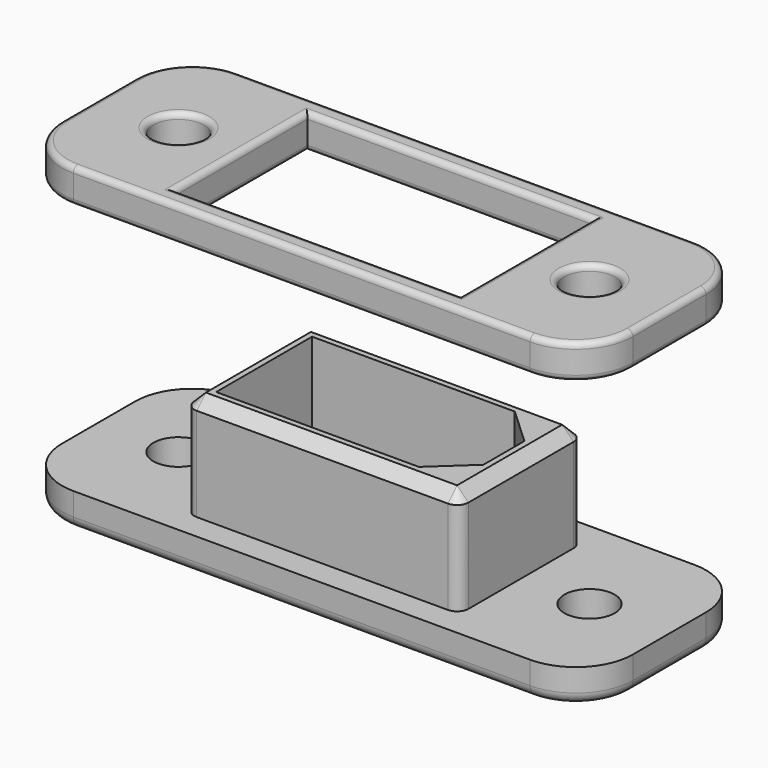
from build123d import *

# Parameters (mm, degrees)
F0_W          = 50
F0_H          = 18
F0_R          = 2.2
F0_W_2        = 21
F0_H_2        = 10.5
F1_DEPTH      = 3
F2_W          = 24
F2_H          = 13.5
F3_DEPTH      = 9.2
F3_DEPTH_BACK = 3
F4_R          = 5
F5_R          = 1
F7_R          = 1
F8_SIZE       = 0.99999
F10_START     = 22
F9_R          = 2.2
F9_W          = 25
F9_H          = 14.5
F10_DEPTH     = 3
F11_R         = 0.5


# Not quite as in the source:
# - a fillet or chamfer is up to 0.001 mm smaller than in the source, because OpenCascade refuses the exact size


with BuildPart() as f1:
    # F0 (on Top) → F1 (new body)
    with BuildSketch(Plane.XY):
        Rectangle(F0_W, F0_H)
        with Locations((-18, 0)):
            Circle(F0_R, mode=Mode.SUBTRACT)
        Rectangle(F0_W_2, F0_H_2, mode=Mode.SUBTRACT)
        with Locations((18, 0)):
            Circle(F0_R, mode=Mode.SUBTRACT)
    extrude(amount=F1_DEPTH)

    # F2 (on face) → F3 (join, two sides)
    with BuildSketch(Plane.XY.offset(3)) as f3_sk:
        Rectangle(F2_W, F2_H)
        Polygon((-10.5, 5.25), (7.25, 5.25), (10.5, 2.25), (10.5, -2.25), (7.25, -5.25), (-10.5, -5.25), align=None, mode=Mode.SUBTRACT)
    extrude(amount=F3_DEPTH)
    extrude(f3_sk.sketch, amount=-F3_DEPTH_BACK)

    # F4
    f4_edges = [f1.edges().sort_by_distance(p)[0] for p in [
        (-25, -9, 1.5),
        (-25, 9, 1.5),
        (25, 9, 1.5),
        (25, -9, 1.5),
    ]]
    fillet(f4_edges, radius=F4_R)

    # F5
    f5_edges = [f1.edges().sort_by_distance(p)[0] for p in [
        (0, 9, 0),
    ]]
    fillet(f5_edges, radius=F5_R)

    # F7
    f7_edges = [f1.edges().sort_by_distance(p)[0] for p in [
        (-12, 6.75, 7.6),
        (12, 6.75, 7.6),
        (12, -6.75, 7.6),
        (-12, -6.75, 7.6),
    ]]
    fillet(f7_edges, radius=F7_R)

    # F8 (size 1 in the source; OpenCascade refuses exactly that, so slightly less here)
    f8_edges = [f1.edges().sort_by_distance(p)[0] for p in [
        (0, 6.75, 12.2),
        (-11.707107, 6.457107, 12.2),
        (-12, 0, 12.2),
    ]]
    chamfer(f8_edges, length=F8_SIZE)


with BuildPart() as f10:
    # F9 (on face) → F10 (new body)
    with BuildSketch(Plane.XY.offset(3).offset(F10_START)):
        with BuildLine():
            ThreePointArc((25, 4), (23.5355339059, 7.5355339059), (20, 9))
            Line((20, 9), (-20, 9))
            ThreePointArc((-20, 9), (-23.5355339059, 7.5355339059), (-25, 4))
            Line((-25, 4), (-25, -4))
            ThreePointArc((-25, -4), (-23.5355339059, -7.5355339059), (-20, -9))
            Line((-20, -9), (20, -9))
            ThreePointArc((20, -9), (23.5355339059, -7.5355339059), (25, -4))
            Line((25, -4), (25, 4))
        make_face()
        with Locations((-18, 0)):
            Circle(F9_R, mode=Mode.SUBTRACT)
        Rectangle(F9_W, F9_H, mode=Mode.SUBTRACT)
        with Locations((18, 0)):
            Circle(F9_R, mode=Mode.SUBTRACT)
    extrude(amount=F10_DEPTH)

    # F11
    f11_edges = [f10.edges().sort_by_distance(p)[0] for p in [
        (23.535534, 7.535534, 25),
        (0, 9, 25),
        (-23.535534, 7.535534, 25),
        (-25, 0, 25),
        (-23.535534, -7.535534, 25),
        (0, -9, 25),
        (23.535534, -7.535534, 25),
        (25, 0, 25),
        (-20.2, 0, 25),
        (-12.5, 0, 25),
        (0, 7.25, 25),
        (12.5, 0, 25),
        (0, -7.25, 25),
        (15.8, 0, 25),
        (23.535534, 7.535534, 28),
        (0, 9, 28),
        (-23.535534, 7.535534, 28),
        (-25, 0, 28),
        (-23.535534, -7.535534, 28),
        (0, -9, 28),
        (23.535534, -7.535534, 28),
        (25, 0, 28),
        (-20.2, 0, 28),
        (-12.5, 0, 28),
        (0, 7.25, 28),
        (12.5, 0, 28),
        (0, -7.25, 28),
        (15.8, 0, 28),
    ]]
    fillet(f11_edges, radius=F11_R)


solid = Compound([f1.part, f10.part])
